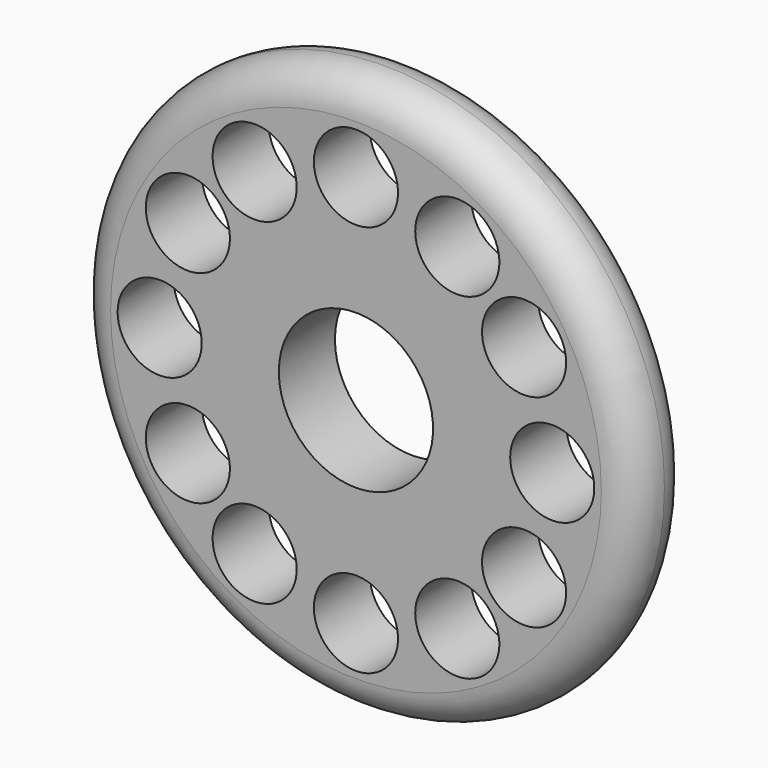
from build123d import *

# Parameters (mm, degrees)
F0_R     = 40
F1_DEPTH = 5
F3_D     = 22
F4_D     = 12
F5_R     = 4.99999


# Not quite as in the source:
# - a fillet or chamfer is up to 0.001 mm smaller than in the source, because OpenCascade refuses the exact size
# - a feature names something its author has since deleted; it is built from what else it names


with BuildPart() as f1:
    # F0 (on Front) → F1 (new body, symmetric)
    with BuildSketch(Plane.XZ):
        Circle(F0_R)
    extrude(amount=F1_DEPTH, both=True)

    # F3 (through all)
    with Locations(Plane.XZ.offset(5)):
        with Locations((0, 0)):
            Hole(F3_D / 2)

    # F4 (through all)
    with Locations(Plane.XZ.offset(5)):
        with Locations((-28, 0), (0, 28), (28, 0), (0, -28), (-23.9821428571, 14.4518796002), (-14.4518796002, 23.9821428571), (14.4518796002, 23.9821428571), (23.9821428571, 14.4518796002), (23.9821428571, -14.4518796002), (-14.4518796002, -23.9821428571), (14.4518796002, -23.9821428571), (-23.9821428571, -14.4518796002)):
            Hole(F4_D / 2)

    # F5 (radius 5 in the source; OpenCascade refuses exactly that, so slightly less here)
    f5_edges = [f1.edges().sort_by_distance(p)[0] for p in [
        (-40, -5, 0),
        (-40, 5, 0),
        (40, 0, 0),
    ]]
    fillet(f5_edges, radius=F5_R)


solid = f1.part
